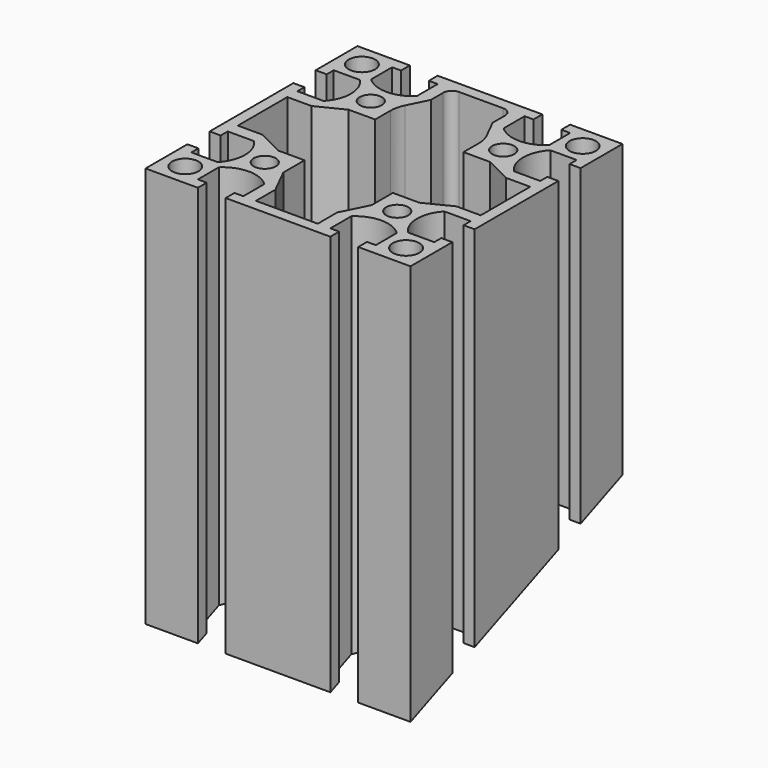
from build123d import *

# Parameters (mm, degrees)
F0_R          = 3
F0_R_2        = 2.5
F1_DEPTH      = 115.678
F2_R          = 2
F3_R          = 7
F6_DEPTH      = 30
F6_DEPTH_BACK = 30
F7_W          = 131.1645284295
F7_H          = 50.7057756186
F8_DEPTH      = 30
F8_DEPTH_BACK = 30


# Not quite as in the source:
# - a feature names something its author has since deleted; it is built from what else it names


with BuildPart() as f1:
    # F0 (on Top) → F1 (new body)
    with BuildSketch(Plane.XY):
        with BuildLine():
            Line((18.15, -30), (30, -30))
            Line((30, -30), (30, -18.15))
            Line((30, -18.15), (27.5, -18.15))
            Line((27.5, -18.15), (27.5, -20.15))
            Line((27.5, -20.15), (21.5477069044, -20.15))
            ThreePointArc((21.5477069044, -20.15), (19.5, -15), (21.5477069044, -9.85))
            Line((21.5477069044, -9.85), (27.5, -9.85))
            Line((27.5, -9.85), (27.5, -11.85))
            Line((27.5, -11.85), (30, -11.85))
            Line((30, -11.85), (30, 11.85))
            Line((30, 11.85), (27.5, 11.85))
            Line((27.5, 11.85), (27.5, 9.85))
            Line((27.5, 9.85), (21.5477069044, 9.85))
            ThreePointArc((21.5477069044, 9.85), (19.5, 15), (21.5477069044, 20.15))
            Line((21.5477069044, 20.15), (27.5, 20.15))
            Line((27.5, 20.15), (27.5, 18.15))
            Line((27.5, 18.15), (30, 18.15))
            Line((30, 18.15), (30, 30))
            Line((30, 30), (18.15, 30))
            Line((18.15, 30), (18.15, 27.5))
            Line((18.15, 27.5), (20.15, 27.5))
            Line((20.15, 27.5), (20.15, 21.5477069044))
            ThreePointArc((20.15, 21.5477069044), (15, 19.5), (9.85, 21.5477069044))
            Line((9.85, 21.5477069044), (9.85, 27.5))
            Line((9.85, 27.5), (11.85, 27.5))
            Line((11.85, 27.5), (11.85, 30))
            Line((11.85, 30), (-11.85, 30))
            Line((-11.85, 30), (-11.85, 27.5))
            Line((-11.85, 27.5), (-9.85, 27.5))
            Line((-9.85, 27.5), (-9.85, 21.5477069044))
            ThreePointArc((-9.85, 21.5477069044), (-15, 19.5), (-20.15, 21.5477069044))
            Line((-20.15, 21.5477069044), (-20.15, 27.5))
            Line((-20.15, 27.5), (-18.15, 27.5))
            Line((-18.15, 27.5), (-18.15, 30))
            Line((-18.15, 30), (-30, 30))
            Line((-30, 30), (-30, 18.15))
            Line((-30, 18.15), (-27.5, 18.15))
            Line((-27.5, 18.15), (-27.5, 20.15))
            Line((-27.5, 20.15), (-21.5477069044, 20.15))
            ThreePointArc((-21.5477069044, 20.15), (-19.5, 15), (-21.5477069044, 9.85))
            Line((-21.5477069044, 9.85), (-27.5, 9.85))
            Line((-27.5, 9.85), (-27.5, 11.85))
            Line((-27.5, 11.85), (-30, 11.85))
            Line((-30, 11.85), (-30, -11.85))
            Line((-30, -11.85), (-27.5, -11.85))
            Line((-27.5, -11.85), (-27.5, -9.85))
            Line((-27.5, -9.85), (-21.5477069044, -9.85))
            ThreePointArc((-21.5477069044, -9.85), (-19.5, -15), (-21.5477069044, -20.15))
            Line((-21.5477069044, -20.15), (-27.5, -20.15))
            Line((-27.5, -20.15), (-27.5, -18.15))
            Line((-27.5, -18.15), (-30, -18.15))
            Line((-30, -18.15), (-30, -30))
            Line((-30, -30), (-18.15, -30))
            Line((-18.15, -30), (-18.15, -27.5))
            Line((-18.15, -27.5), (-20.15, -27.5))
            Line((-20.15, -27.5), (-20.15, -21.5477069044))
            ThreePointArc((-20.15, -21.5477069044), (-15, -19.5), (-9.85, -21.5477069044))
            Line((-9.85, -21.5477069044), (-9.85, -27.5))
            Line((-9.85, -27.5), (-11.85, -27.5))
            Line((-11.85, -27.5), (-11.85, -30))
            Line((-11.85, -30), (11.85, -30))
            Line((11.85, -30), (11.85, -27.5))
            Line((11.85, -27.5), (9.85, -27.5))
            Line((9.85, -27.5), (9.85, -21.5477069044))
            ThreePointArc((9.85, -21.5477069044), (15, -19.5), (20.15, -21.5477069044))
            Line((20.15, -21.5477069044), (20.15, -27.5))
            Line((20.15, -27.5), (18.15, -27.5))
            Line((18.15, -27.5), (18.15, -30))
        make_face()
        with Locations((-25, -25)):
            Circle(F0_R, mode=Mode.SUBTRACT)
        with Locations((-15, -15)):
            Circle(F0_R_2, mode=Mode.SUBTRACT)
        with Locations((25, -25)):
            Circle(F0_R, mode=Mode.SUBTRACT)
        with Locations((15, -15)):
            Circle(F0_R_2, mode=Mode.SUBTRACT)
        with Locations((-25, 25)):
            Circle(F0_R, mode=Mode.SUBTRACT)
        with Locations((-15, 15)):
            Circle(F0_R_2, mode=Mode.SUBTRACT)
        Polygon((-7, 22), (-7, 27.5), (0, 27.5), (7, 27.5), (7, 22), (10, 16), (10, 10), (16, 10), (22, 7), (27.5, 7), (27.5, 0), (27.5, -7), (22, -7), (16, -10), (10, -10), (10, -16), (7, -22), (7, -27.5), (0, -27.5), (-7, -27.5), (-7, -22), (-10, -16), (-10, -10), (-16, -10), (-22, -7), (-27.5, -7), (-27.5, 0), (-27.5, 7), (-22, 7), (-16, 10), (-10, 10), (-10, 16), align=None, mode=Mode.SUBTRACT)
        with Locations((15, 15)):
            Circle(F0_R_2, mode=Mode.SUBTRACT)
        with Locations((25, 25)):
            Circle(F0_R, mode=Mode.SUBTRACT)
    extrude(amount=F1_DEPTH)

    # F2
    f2_edges = [f1.edges().sort_by_distance(p)[0] for p in [
        (-7, 27.5, 57.839),
        (7, 27.5, 57.839),
    ]]
    fillet(f2_edges, radius=F2_R)

    # F3
    f3_edges = [f1.edges().sort_by_distance(p)[0] for p in [
        (-10, 16, 57.839),
        (10, 16, 57.839),
    ]]
    fillet(f3_edges, radius=F3_R)

    # F5 (on Right) → F6 (cut, two sides)
    with BuildSketch(Plane.YZ) as f6_sk:
        Polygon((214.5999793503, -135.2321386172), (130.9673605882, 66.674863855), (-30, 0), (53.6326187621, -201.9070024722), align=None)
        Polygon((30, 115.678), (-2.0081647111, 192.9525453523), (-162.3392477394, 126.541236292), (-130.3310830283, 49.2666909397), align=None)
    extrude(amount=-F6_DEPTH, mode=Mode.SUBTRACT)
    extrude(f6_sk.sketch, amount=F6_DEPTH_BACK, mode=Mode.SUBTRACT)

    # F7 (on Right) → F8 (cut, two sides)
    with BuildSketch(Plane.YZ) as f8_sk:
        with Locations((35.5822642148, 116.1780740669)):
            Rectangle(F7_W, F7_H)
    extrude(amount=F8_DEPTH, mode=Mode.SUBTRACT)
    extrude(f8_sk.sketch, amount=-F8_DEPTH_BACK, mode=Mode.SUBTRACT)


solid = f1.part
